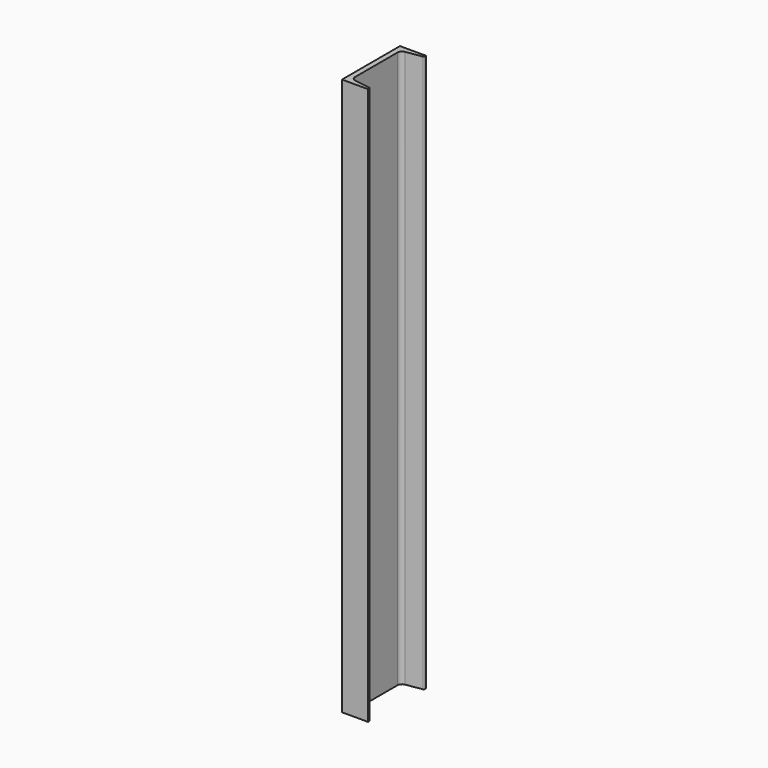
from build123d import *

# Parameters (mm, degrees)
F1_DEPTH = 1171.575


# Not quite as in the source:
# - ends of sketch curves that miss each other by under 0.0002 mm in the source are joined


with BuildPart() as f1:
    # F0 (on Top) → F1 (new body)
    with BuildSketch(Plane.XY):
        with BuildLine():
            Line((-27.3939, 76.2), (-27.3939, -76.2))
            Line((-27.3939, -76.2), (27.3939, -76.2))
            Line((27.3939, -76.2), (27.3939, -73.2072196))
            ThreePointArc((27.3939, -73.2072196), (26.7702370991, -71.514649446), (25.1974607678, -70.6314033014))
            Line((25.1974607678, -70.6314033014), (-8.2739484, -65.2759934))
            ThreePointArc((-8.2739484, -65.2759934), (-14.0168334338, -62.0508920476), (-16.2941, -55.870602))
            Line((-16.2941, -55.870602), (-16.2941, 55.870602))
            ThreePointArc((-16.2941, 55.870602), (-14.0168334338, 62.0508920476), (-8.2739456541, 65.275976238))
            Line((-8.2739456541, 65.275976238), (25.1974604, 70.6314056))
            ThreePointArc((25.1974604, 70.6314056), (26.7702370991, 71.514649446), (27.3939, 73.2072196))
            Line((27.3939, 73.2072196), (27.3939, 76.2))
            Line((27.3939, 76.2), (-27.3939, 76.2))
        make_face()
    extrude(amount=F1_DEPTH)


solid = f1.part
